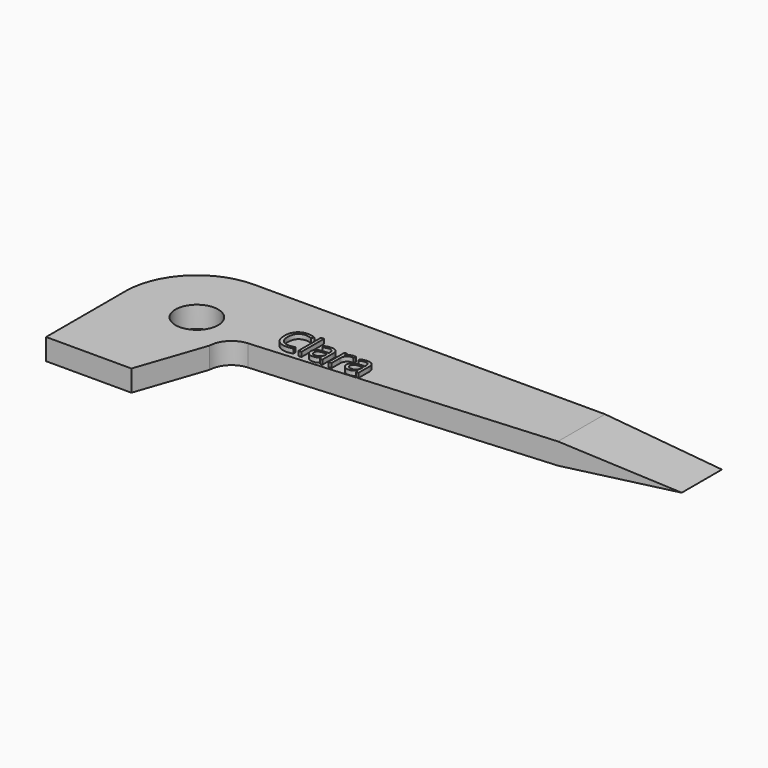
from build123d import *

# Parameters (mm, degrees)
F1_DEPTH     = 2.38125
F2_R         = 2.38125
F3_DEPTH     = 2.38125
F5_DEPTH     = 25.4
F6_TEXT_SIZE = 4.1650069633
F7_DEPTH     = 0.508


# Not quite as in the source:
# - Text() gives the source's letters only with a copy of the font that has no kerning and outlines rounded to 1/6400 em; it was checked with that copy


with BuildPart() as f1:
    # F0 (on Top) → F1 (new body)
    with BuildSketch(Plane.XY):
        with BuildLine():
            Line((60.198, 19.05), (7.9375, 19.05))
            ThreePointArc((7.9375, 19.05), (2.3248399243, 16.7251600757), (0, 11.1125))
            Line((0, 11.1125), (0, 0))
            Line((0, 0), (9.525, 0))
            Line((9.525, 0), (12.1395677624, 7.6374629666))
            ThreePointArc((12.1395677624, 7.6374629666), (12.8398802022, 9.2928209665), (14.4665166472, 10.057478731))
            Line((14.4665166472, 10.057478731), (60.198, 13.4413698688))
            Line((60.198, 13.4413698688), (60.198, 19.05))
        make_face()
    extrude(amount=F1_DEPTH)

    # F2 (on face) → F3 (cut)
    with BuildSketch(Plane.XY.offset(2.38125)):
        with Locations((7.9375, 11.1125)):
            Circle(F2_R)
    extrude(amount=-F3_DEPTH, mode=Mode.SUBTRACT)

    # F4 (on face) → F5 (cut)
    with BuildSketch(Plane(origin=(0, 19.05, 0), x_dir=(-1, 0, 0), z_dir=(0, 1, 0))):
        Polygon((-60.198, 0), (-47.1547567568, 0), (-60.198, 1.190625), align=None)
        Polygon((-60.198, 2.38125), (-60.198, 1.190625), (-47.1547567568, 2.38125), align=None)
    extrude(amount=-F5_DEPTH, mode=Mode.SUBTRACT)

    # F6 (on face) → F7 (join)
    with BuildSketch(Plane.XY.offset(2.38125)):
        with Locations((16.420815041, 10.9381281039)):
            Text('Clara', F6_TEXT_SIZE, font='Open Sans', text_align=(TextAlign.LEFT, TextAlign.BOTTOM))
    extrude(amount=F7_DEPTH)


solid = f1.part
